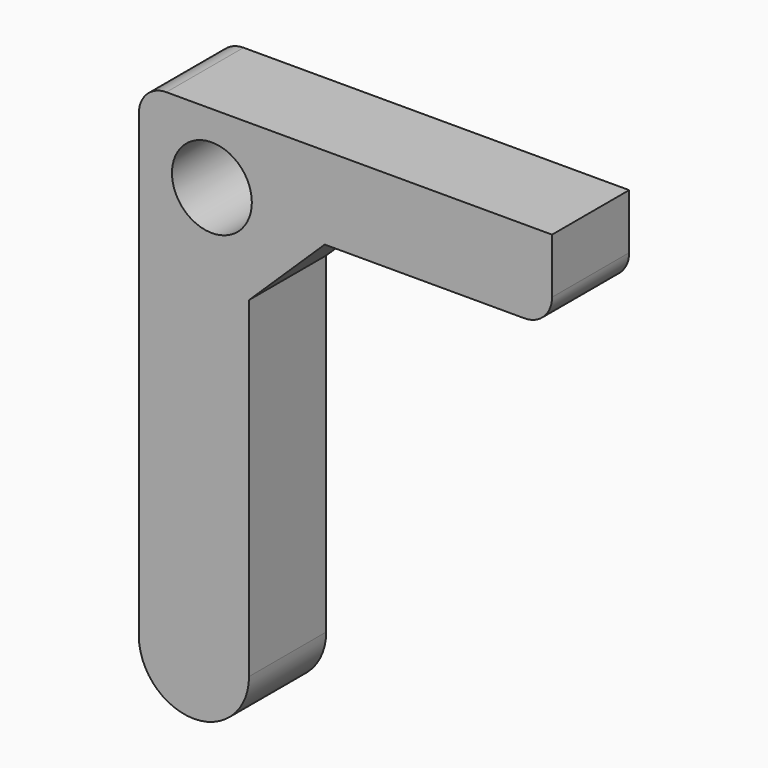
from build123d import *

# Parameters (mm, degrees)
F1_DEPTH    = 8.89
F2_R        = 3.683
F3_DEPTH    = 13.208
F4_R        = 2.54
F5_T1_DEPTH = 38.1
F6_T1_DEPTH = 47.4109630585


# Not quite as in the source:
# - a fillet or chamfer that OpenCascade refuses, or shapes differently, is made with other operations: its cross-section is extruded or revolved along the edge and cut away or added


with BuildPart() as f1:
    # F0 (on Front) → F1 (new body)
    with BuildSketch(Plane.XZ):
        Polygon((0, 50.8), (0, 0), (10.16, 0), (10.16, 36.405056715), (10.16, 43.18), (17.1377565712, 43.18), (38.1, 43.18), (38.1, 50.8), align=None)
        Polygon((10.16, 43.18), (10.16, 36.405056715), (17.1377565712, 43.18), align=None)
    extrude(amount=F1_DEPTH)

    # F2 (on Front) → F3 (cut)
    with BuildSketch(Plane.XZ):
        with Locations((6.7352303304, 44.409301132)):
            Circle(F2_R)
    extrude(amount=F3_DEPTH, mode=Mode.SUBTRACT)

    # F4
    f4_edges = [f1.edges().sort_by_distance(p)[0] for p in [
        (0, -4.445, 50.8),
        (38.1, -4.445, 43.18),
    ]]
    fillet(f4_edges, radius=F4_R)

    # F5: fillet of radius 5.842 on 2 edges, made by hand

    # F5_s2 → F5_t1 (cut)
    with BuildSketch(Plane.XZ.offset(-14.605)):
        with BuildLine():
            ThreePointArc((0, 5.842), (1.7110821843, 1.7110821843), (5.842, 0))
            Line((5.842, 0), (0, 0))
            Line((0, 0), (0, 5.842))
        make_face()
        with BuildLine():
            ThreePointArc((4.318, 0), (8.4489178157, 1.7110821843), (10.16, 5.842))
            Line((10.16, 5.842), (10.16, 0))
            Line((10.16, 0), (4.318, 0))
        make_face()
    extrude(amount=F5_T1_DEPTH, mode=Mode.SUBTRACT)

    # F6: fillet of radius 5.08 on 1 edges, made by hand

    # F6_s2 → F6_t1 (cut)
    with BuildSketch(Plane.XZ.offset(-19.2604815292)):
        with BuildLine():
            ThreePointArc((0, 5.8419882424), (5.08, 0.7619984664), (10.16, 5.8419882424))
            ThreePointArc((10.16, 5.8419882424), (8.710066706, 1.9898948547), (5.08, 0.0499088405))
            ThreePointArc((5.08, 0.0499088405), (1.449933294, 1.9898948547), (0, 5.8419882424))
        make_face()
    extrude(amount=F6_T1_DEPTH, mode=Mode.SUBTRACT)


solid = f1.part
